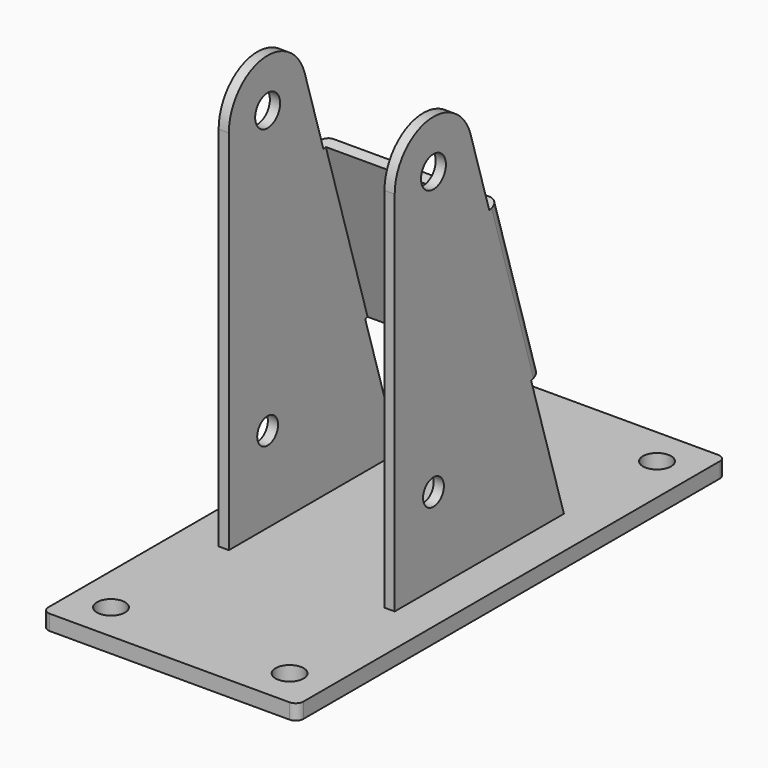
from build123d import *

# Parameters (mm, degrees)
F0_R          = 5.1
F0_R_2        = 6.1
F1_DEPTH      = 34.5
F2_R          = 4
F3_T          = 4
F4_DEPTH      = 50
F4_DEPTH_BACK = 50
F5_R          = 3
F7_D          = 11
F9_D          = 6.8


# Not quite as in the source:
# - ends of sketch curves that miss each other by under 0.0002 mm in the source are joined
# - a shell that OpenCascade refuses in one call is made with other operations: the cavity is built on its own and cut out
# - a feature names something its author has since deleted; it is built from what else it names


with BuildPart() as f1:
    # F0 (on Right) → F1 (new body, symmetric)
    with BuildSketch(Plane.YZ):
        with BuildLine():
            Line((1.885386, -78.484767), (45, -78.484767))
            Line((45, -78.484767), (28.944748, -25.970405))
            Line((28.944748, -25.970405), (33.917533, -24.450072))
            Line((33.917533, -24.450072), (13.451514, 42.49126))
            Line((13.451514, 42.49126), (8.478729, 40.970928))
            Line((8.478729, 40.970928), (-0.714257, 71.03983))
            ThreePointArc((-0.714257, 71.03983), (-21.6924256797, 84.2760694236), (-37.884047, 65.484768))
            Line((-37.884047, 65.484768), (-37.884047, -78.484767))
            Line((-37.884047, -78.484767), (-3.771468, -78.484767))
            Line((-3.771468, -78.484767), (1.885386, -78.484767))
        make_face()
        with Locations((-18.884047, -44.984767)):
            Circle(F0_R, mode=Mode.SUBTRACT)
        with Locations((-18.893362, 65.515233)):
            Circle(F0_R_2, mode=Mode.SUBTRACT)
    extrude(amount=F1_DEPTH, both=True)

    # F2
    f2_edges = [f1.edges().sort_by_distance(p)[0] for p in [
        (-34.5, 23.684523, 9.020594),
        (34.5, 23.684523, 9.020594),
    ]]
    fillet(f2_edges, radius=F2_R)

    # F3: shell of thickness 4, made by hand


with BuildPart() as f3_core1:
    # F3_t2: copy of F1
    add(f1.part)

    # the walls: a layer under each face that stays
    f3_faces = [f3_core1.faces().sort_by_distance(p)[0] for p in [
        (-34.5, 3.5579765, 3.0000004813),
        (0, 23.6845235, 9.020594),
        (34.5, 3.5579765, 3.0000004813),
    ]]
    thicken(f3_faces, amount=-F3_T, mode=Mode.SUBTRACT)


with BuildPart() as f1_1:
    add(f1.part)

    # what is left inside the walls is the cavity
    f3_cavity = [f3_core1.part.solids().sort_by_distance(p)[0] for p in [
        (-30.46, 3.557976, -24.161589),
    ]]
    add(f3_cavity, mode=Mode.SUBTRACT)

    # F0 (on Right) → F4 (join, two sides)
    with BuildSketch(Plane.YZ) as f4_sk:
        Polygon((-105, -84.484767), (105, -84.484767), (105, -78.484767), (45, -78.484767), (1.885386, -78.484767), (-3.771468, -78.484767), (-37.884047, -78.484767), (-105, -78.484767), align=None)
    extrude(amount=F4_DEPTH)
    extrude(f4_sk.sketch, amount=-F4_DEPTH_BACK)

    # F5
    f5_edges = [f1_1.edges().sort_by_distance(p)[0] for p in [
        (-50, -105, -81.484767),
        (50, -105, -81.484767),
        (50, 105, -81.484767),
        (-50, 105, -81.484767),
    ]]
    fillet(f5_edges, radius=F5_R)

    # F7 (through all)
    with Locations(Plane.XY.offset(-78.484767)):
        with Locations((-35, 90), (-35, -90), (35, -90), (35, 90)):
            Hole(F7_D / 2)

    # F9 (through all)
    with Locations(Plane(origin=(0, 24.1820677637, 7.3932000384), x_dir=(-1, 0, 0), z_dir=(0, 0.9563047562, 0.2923717041))):
        with Locations((0, 22.7017519629), (0, -19.2982480371)):
            Hole(F9_D / 2)


solid = f1_1.part
